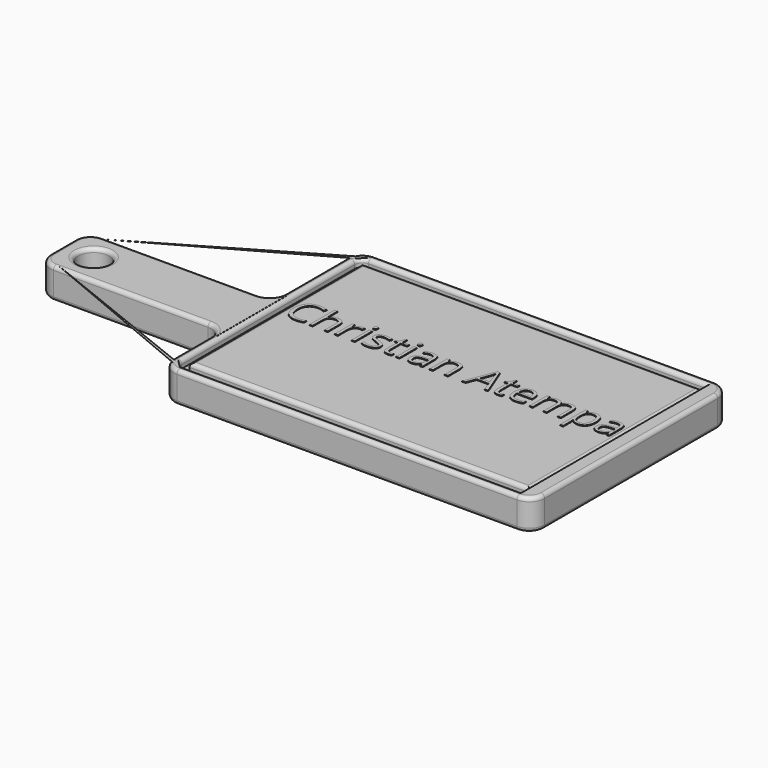
from build123d import *

# Parameters (mm, degrees)
F0_W         = 152.4
F0_H         = 50.8
F1_DEPTH     = 25.4
F2_R         = 12.7
F3_DEPTH     = 25.4
F5_DEPTH     = 6.35
F6_R         = 6.35
F7_R         = 12.7
F8_R         = 3.17499
F9_TEXT_SIZE = 33.9258400931
F10_DEPTH    = 0.508


# Not quite as in the source:
# - a fillet or chamfer is up to 0.001 mm smaller than in the source, because OpenCascade refuses the exact size
# - Text() gives the source's letters only with a copy of the font that has no kerning and outlines rounded to 1/6400 em; it was checked with that copy


with BuildPart() as f1:
    # F0 (on Top) → F1 (new body)
    with BuildSketch(Plane.XY):
        Polygon((0, 63.5), (0, 0), (304.8, 0), (304.8, 203.2), (0, 203.2), (0, 114.3), align=None)
        with Locations((-76.2, 88.9)):
            Rectangle(F0_W, F0_H)
    extrude(amount=F1_DEPTH)

    # F2 (on face) → F3 (cut)
    with BuildSketch(Plane.XY.offset(25.4)):
        with Locations((-127, 88.9)):
            Circle(F2_R)
    extrude(amount=-F3_DEPTH, mode=Mode.SUBTRACT)

    # F4 (on face) → F5 (cut)
    with BuildSketch(Plane.XY.offset(25.4)):
        Polygon((6.349998188, 63.5), (6.349998188, 6.349998188), (298.450001812, 6.349998188), (298.450001812, 196.850001812), (6.349998188, 196.850001812), (6.349998188, 114.3), align=None)
        Polygon((12.699998188, 63.5), (12.699998188, 114.3), (12.699998188, 190.500001812), (292.100001812, 190.500001812), (292.100001812, 12.699998188), (12.699998188, 12.699998188), align=None, mode=Mode.SUBTRACT)
    extrude(amount=-F5_DEPTH, mode=Mode.SUBTRACT)

    # F6
    f6_edges = [f1.edges().sort_by_distance(p)[0] for p in [
        (6.349998, 196.850002, 22.225),
        (298.450002, 196.850002, 22.225),
        (298.450002, 6.349998, 22.225),
        (6.349998, 6.349998, 22.225),
    ]]
    fillet(f6_edges, radius=F6_R)

    # F7
    f7_edges = [f1.edges().sort_by_distance(p)[0] for p in [
        (0, 0, 12.7),
        (-152.4, 63.5, 12.7),
        (0, 203.2, 12.7),
        (-152.4, 114.3, 12.7),
        (304.8, 203.2, 12.7),
        (304.8, 0, 12.7),
        (0, 63.5, 12.7),
        (0, 114.3, 12.7),
    ]]
    fillet(f7_edges, radius=F7_R)

    # F8 (radius 3.175 in the source; OpenCascade refuses exactly that, so slightly less here)
    f8_edges = [f1.edges().sort_by_distance(p)[0] for p in [
        (152.4, 12.699998, 25.4),
        (12.699998, 101.6, 25.4),
        (152.4, 190.500002, 25.4),
        (292.100002, 101.6, 25.4),
        (0, 31.75, 25.4),
        (-3.719744, 59.780256, 25.4),
        (3.719744, 3.719744, 25.4),
        (-76.2, 63.5, 25.4),
        (152.4, 0, 25.4),
        (-148.680256, 67.219744, 25.4),
        (301.080256, 3.719744, 25.4),
        (-152.4, 88.9, 25.4),
        (304.8, 101.6, 25.4),
        (-148.680256, 110.580256, 25.4),
        (301.080256, 199.480256, 25.4),
        (-76.2, 114.3, 25.4),
        (152.4, 203.2, 25.4),
        (-3.719744, 118.019744, 25.4),
        (3.719744, 199.480256, 25.4),
        (0, 158.75, 25.4),
        (152.4, 6.349998, 25.4),
        (8.20987, 8.20987, 25.4),
        (296.59013, 8.20987, 25.4),
        (6.349998, 101.6, 25.4),
        (298.450002, 101.6, 25.4),
        (8.20987, 194.99013, 25.4),
        (296.59013, 194.99013, 25.4),
        (152.4, 196.850002, 25.4),
        (-139.7, 88.9, 25.4),
        (0, 31.75, 0),
        (-3.719744, 59.780256, 0),
        (3.719744, 3.719744, 0),
        (-76.2, 63.5, 0),
        (152.4, 0, 0),
        (-148.680256, 67.219744, 0),
        (301.080256, 3.719744, 0),
        (-152.4, 88.9, 0),
        (304.8, 101.6, 0),
        (-148.680256, 110.580256, 0),
        (301.080256, 199.480256, 0),
        (-76.2, 114.3, 0),
        (152.4, 203.2, 0),
        (-3.719744, 118.019744, 0),
        (3.719744, 199.480256, 0),
        (0, 158.75, 0),
        (-139.7, 88.9, 0),
    ]]
    fillet(f8_edges, radius=F8_R)

    # F9 (on face) → F10 (join)
    with BuildSketch(Plane.XY.offset(25.4)):
        with Locations((15.874998188, 101.6)):
            Text('Christian Atempa', F9_TEXT_SIZE, font='Open Sans', text_align=(TextAlign.LEFT, TextAlign.BOTTOM))
    extrude(amount=F10_DEPTH)


solid = f1.part
